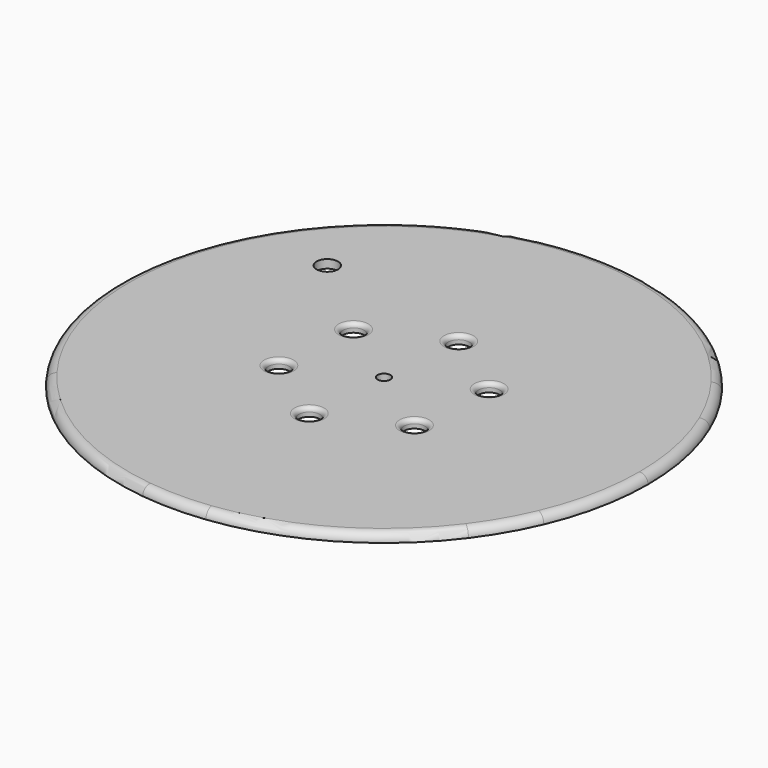
from build123d import *

# Parameters (mm, degrees)
F0_R     = 2.5
F0_R_2   = 2.5423106838
F1_DEPTH = 2
F2_R     = 1
F3_R     = 1
F4_R     = 1.99999
F5_R     = 1.5
F6_DEPTH = 2


# Not quite as in the source:
# - a fillet or chamfer is up to 0.001 mm smaller than in the source, because OpenCascade refuses the exact size


with BuildPart() as f1:
    # F0 (on Top) → F1 (new body)
    with BuildSketch(Plane.XY):
        Polygon((-35.0480947162, -37.5), (35.0480947162, -37.5), (50, -28.8675134595), (50, 28.8675134595), (35.0480947162, 37.5), (-35.0480947162, 37.5), (-50, 28.8675134595), (-50, -28.8675134595), align=None)
        with Locations((-1.743114855, -19.9238939618)):
            Circle(F0_R, mode=Mode.SUBTRACT)
        with Locations((-18.1261557407, -8.4523652348)):
            Circle(F0_R, mode=Mode.SUBTRACT)
        with Locations((16.3830408858, -11.471528727)):
            Circle(F0_R, mode=Mode.SUBTRACT)
        with Locations((-36.1640639603, 28.4298043698)):
            Circle(F0_R_2, mode=Mode.SUBTRACT)
        with Locations((-16.3830408858, 11.471528727)):
            Circle(F0_R, mode=Mode.SUBTRACT)
        with Locations((18.1261557407, 8.4523652348)):
            Circle(F0_R, mode=Mode.SUBTRACT)
        with Locations((1.743114855, 19.9238939618)):
            Circle(F0_R, mode=Mode.SUBTRACT)
        Polygon((-50, -37.5), (-35.0480947162, -37.5), (-50, -28.8675134595), align=None)
        Polygon((-50, 37.5), (-50, 28.8675134595), (-35.0480947162, 37.5), align=None)
        Polygon((35.0480947162, 37.5), (50, 28.8675134595), (50, 37.5), align=None)
        Polygon((35.0480947162, -37.5), (50, -37.5), (50, -28.8675134595), align=None)
        Polygon((-35.0480947162, 37.5), (35.0480947162, 37.5), (0, 57.735026919), align=None)
        with BuildLine():
            Line((50, 28.8675134595), (50, -28.8675134595))
            Line((50, -28.8675134595), (57.4759526419, -24.5512701892))
            ThreePointArc((57.4759526419, -24.5512701892), (61.2311074541, -12.530023142), (62.5, 0))
            ThreePointArc((62.5, 0), (61.2311074541, 12.530023142), (57.4759526419, 24.5512701892))
            Line((57.4759526419, 24.5512701892), (50, 28.8675134595))
        make_face()
        with BuildLine():
            Line((35.0480947162, 37.5), (50, 37.5))
            ThreePointArc((50, 37.5), (31.25, 54.1265877365), (7.4759526419, 62.0512701892))
            Line((7.4759526419, 62.0512701892), (0, 57.735026919))
            Line((0, 57.735026919), (35.0480947162, 37.5))
        make_face()
        with BuildLine():
            Line((0, 57.735026919), (7.4759526419, 62.0512701892))
            ThreePointArc((7.4759526419, 62.0512701892), (0, 62.5), (-7.4759526419, 62.0512701892))
            Line((-7.4759526419, 62.0512701892), (0, 57.735026919))
        make_face()
        with BuildLine():
            Line((50, -28.8675134595), (50, -37.5))
            ThreePointArc((50, -37.5), (54.1265877365, -31.25), (57.4759526419, -24.5512701892))
            Line((57.4759526419, -24.5512701892), (50, -28.8675134595))
        make_face()
        with BuildLine():
            ThreePointArc((7.4759526419, -62.0512701892), (31.25, -54.1265877365), (50, -37.5))
            Line((50, -37.5), (35.0480947162, -37.5))
            Line((35.0480947162, -37.5), (0, -57.735026919))
            Line((0, -57.735026919), (7.4759526419, -62.0512701892))
        make_face()
        Polygon((0, -57.735026919), (35.0480947162, -37.5), (-35.0480947162, -37.5), align=None)
        with BuildLine():
            Line((0, -57.735026919), (-35.0480947162, -37.5))
            Line((-35.0480947162, -37.5), (-50, -37.5))
            ThreePointArc((-50, -37.5), (-31.25, -54.1265877365), (-7.4759526419, -62.0512701892))
            Line((-7.4759526419, -62.0512701892), (0, -57.735026919))
        make_face()
        with BuildLine():
            ThreePointArc((-57.4759526419, -24.5512701892), (-54.1265877365, -31.25), (-50, -37.5))
            Line((-50, -37.5), (-50, -28.8675134595))
            Line((-50, -28.8675134595), (-57.4759526419, -24.5512701892))
        make_face()
        with BuildLine():
            Line((-57.4759526419, -24.5512701892), (-50, -28.8675134595))
            Line((-50, -28.8675134595), (-50, 28.8675134595))
            Line((-50, 28.8675134595), (-57.4759526419, 24.5512701892))
            ThreePointArc((-57.4759526419, 24.5512701892), (-62.5, 0), (-57.4759526419, -24.5512701892))
        make_face()
        with BuildLine():
            ThreePointArc((-7.4759526419, -62.0512701892), (0, -62.5), (7.4759526419, -62.0512701892))
            Line((7.4759526419, -62.0512701892), (0, -57.735026919))
            Line((0, -57.735026919), (-7.4759526419, -62.0512701892))
        make_face()
        with BuildLine():
            Line((-57.4759526419, 24.5512701892), (-50, 28.8675134595))
            Line((-50, 28.8675134595), (-50, 37.5))
            ThreePointArc((-50, 37.5), (-54.1265877365, 31.25), (-57.4759526419, 24.5512701892))
        make_face()
        with BuildLine():
            Line((-50, 37.5), (-35.0480947162, 37.5))
            Line((-35.0480947162, 37.5), (0, 57.735026919))
            Line((0, 57.735026919), (-7.4759526419, 62.0512701892))
            ThreePointArc((-7.4759526419, 62.0512701892), (-31.25, 54.1265877365), (-50, 37.5))
        make_face()
        with BuildLine():
            Line((50, 37.5), (50, 28.8675134595))
            Line((50, 28.8675134595), (57.4759526419, 24.5512701892))
            ThreePointArc((57.4759526419, 24.5512701892), (54.1265877365, 31.25), (50, 37.5))
        make_face()
    extrude(amount=F1_DEPTH)

    # F2
    f2_edges = [f1.edges().sort_by_distance(p)[0] for p in [
        (-4.243115, -19.923894, 2),
    ]]
    fillet(f2_edges, radius=F2_R)

    # F3
    f3_edges = [f1.edges().sort_by_distance(p)[0] for p in [
        (-20.626156, -8.452365, 2),
        (-18.883041, 11.471529, 2),
        (-0.756885, 19.923894, 2),
        (15.626156, 8.452365, 2),
        (13.883041, -11.471529, 2),
    ]]
    fillet(f3_edges, radius=F3_R)

    # F4 (radius 2 in the source; OpenCascade refuses exactly that, so slightly less here)
    f4_edges = [f1.edges().sort_by_distance(p)[0] for p in [
        (-57.475953, -24.55127, 2),
    ]]
    fillet(f4_edges, radius=F4_R)

    # F5 (on face) → F6 (cut)
    with BuildSketch(Plane.XY.offset(2)):
        Circle(F5_R)
    extrude(amount=-F6_DEPTH, mode=Mode.SUBTRACT)


solid = f1.part
